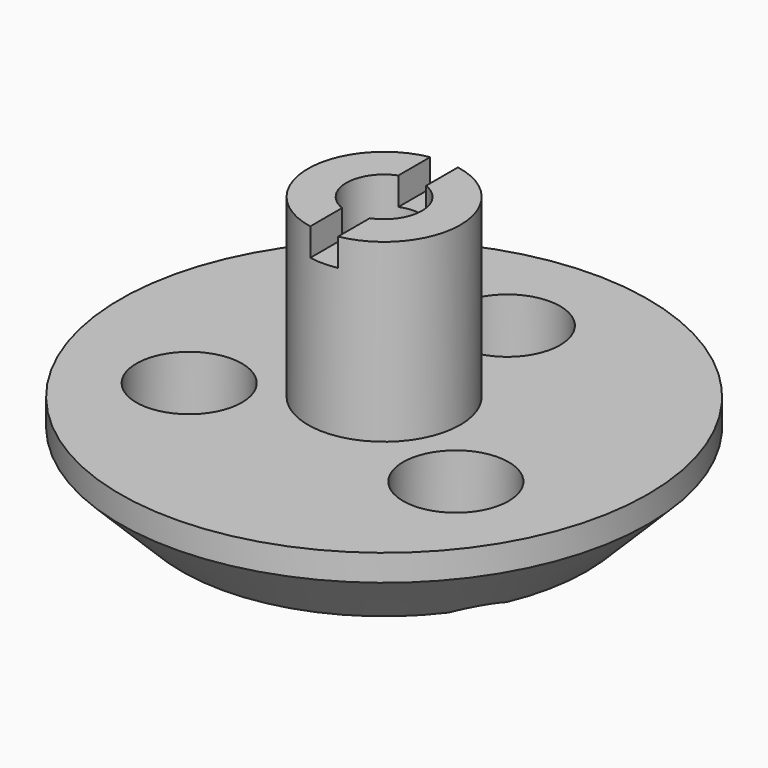
from build123d import *

# Parameters (mm, degrees)
F0_R     = 19.05
F0_R_2   = 3.81
F0_R_3   = 5.4991
F1_DEPTH = 6.35
F0_R_4   = 2.7305
F2_DEPTH = 19.05
F4_DEPTH = 2


# Not quite as in the source:
# - a fillet or chamfer that OpenCascade refuses, or shapes differently, is made with other operations: its cross-section is extruded or revolved along the edge and cut away or added


with BuildPart() as f1:
    # F0 (on Top) → F1 (new body)
    with BuildSketch(Plane.XY):
        Circle(F0_R)
        with Locations((-9.6237072996, -5.55625)):
            Circle(F0_R_2, mode=Mode.SUBTRACT)
        with Locations((9.6237072996, -5.55625)):
            Circle(F0_R_2, mode=Mode.SUBTRACT)
        Circle(F0_R_3, mode=Mode.SUBTRACT)
        with Locations((0, 11.1125)):
            Circle(F0_R_2, mode=Mode.SUBTRACT)
    extrude(amount=F1_DEPTH)

    # F0 (on Top) → F2 (join)
    with BuildSketch(Plane.XY):
        Circle(F0_R_3)
        Circle(F0_R_4, mode=Mode.SUBTRACT)
    extrude(amount=F2_DEPTH)

    # F3 (on face) → F4 (cut)
    with BuildSketch(Plane.XY.offset(19.05)):
        with BuildLine():
            Line((1, 2.5407932324), (1, 5.4074116553))
            ThreePointArc((1, 5.4074116553), (0, 5.4991), (-1, 5.4074116553))
            Line((-1, 5.4074116553), (-1, 2.5407932324))
            ThreePointArc((-1, 2.5407932324), (0, 2.7305), (1, 2.5407932324))
        make_face()
        with BuildLine():
            Line((1, -5.4074116553), (1, -2.5407932324))
            ThreePointArc((1, -2.5407932324), (0, -2.7305), (-1, -2.5407932324))
            Line((-1, -2.5407932324), (-1, -5.4074116553))
            ThreePointArc((-1, -5.4074116553), (0, -5.4991), (1, -5.4074116553))
        make_face()
    extrude(amount=-F4_DEPTH, mode=Mode.SUBTRACT)

    # F5: chamfer of 4.445 on 1 edges, made by hand

    # F5_s1 → F5_t2 (revolve, cut)
    with BuildSketch(Plane.XZ):
        Polygon((19.05, 4.445), (14.605, 0), (19.05, 0), align=None)
    revolve(axis=Axis((0, 0, 0), (0, 0, 1)), mode=Mode.SUBTRACT)


solid = f1.part
